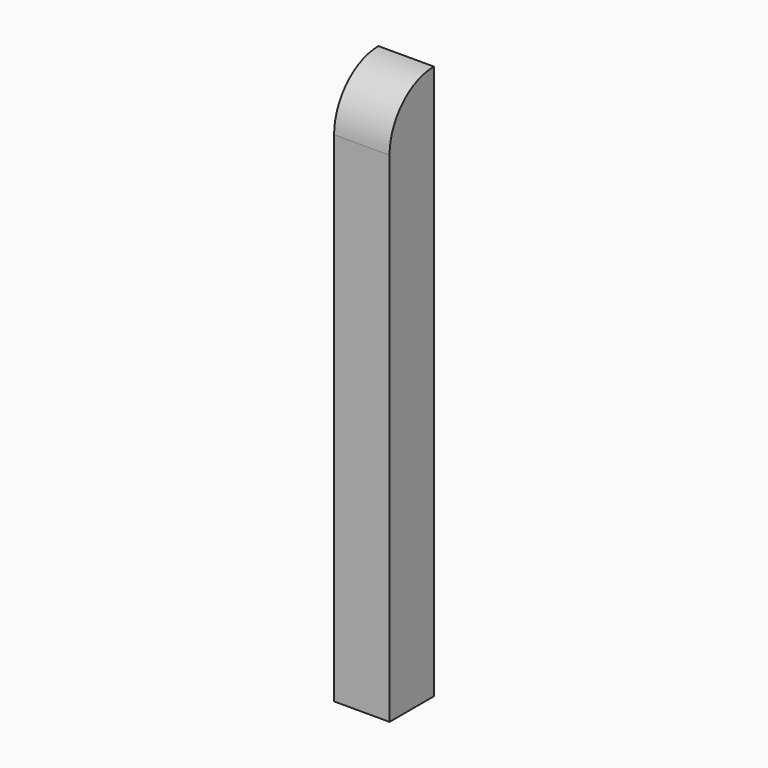
from build123d import *

# Parameters (mm, degrees)
F0_W     = 5
F0_H     = 5
F1_DEPTH = 50
F2_R     = 4.99999


# Not quite as in the source:
# - a fillet or chamfer is up to 0.001 mm smaller than in the source, because OpenCascade refuses the exact size


with BuildPart() as f1:
    # F0 (on Top) → F1 (new body)
    with BuildSketch(Plane.XY):
        Rectangle(F0_W, F0_H)
    extrude(amount=F1_DEPTH)

    # F2 (radius 5 in the source; OpenCascade refuses exactly that, so slightly less here)
    f2_edges = [f1.edges().sort_by_distance(p)[0] for p in [
        (0, -2.5, 50),
    ]]
    fillet(f2_edges, radius=F2_R)


solid = f1.part
